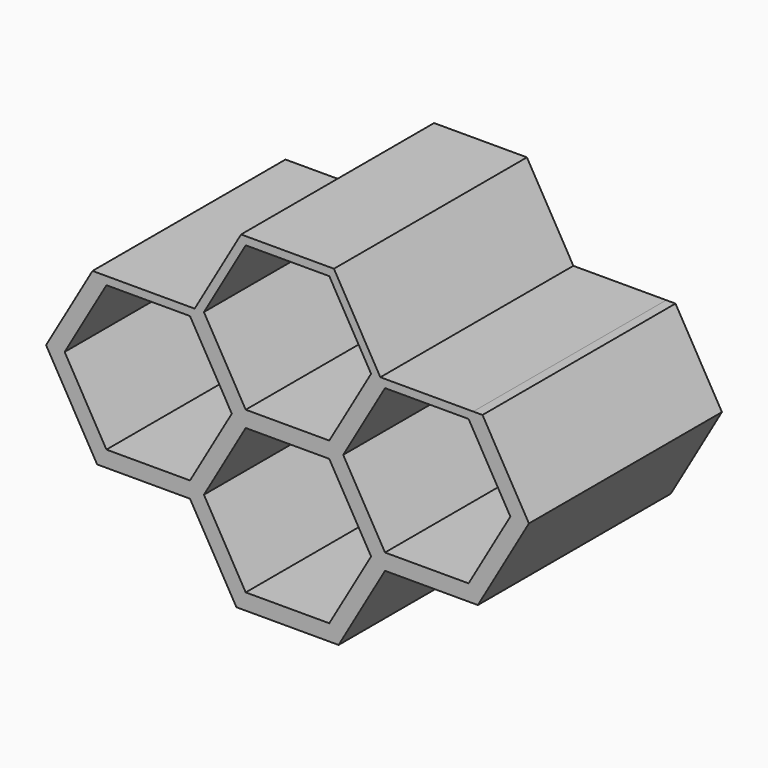
from build123d import *

# Parameters (mm, degrees)
F1_DEPTH = 12.7
F2_DEPTH = 95.25


# Not quite as in the source:
# - a feature names something its author has since deleted; it is built from what else it names


with BuildPart() as f1:
    # F0 (on Front) → F1 (new body)
    with BuildSketch(Plane.XZ):
        Polygon((142.3687008922, 35.0424993012), (105.7069587986, 35.0424993011), (87.3760877519, 3.2924993012), (105.7069587986, -28.4575006988), (142.3687008922, -28.4575006988), (160.6995719389, 3.2924993012), align=None)
        Polygon((107.5400459033, -25.2825006989), (91.0422619612, 3.2924993011), (107.5400459033, 31.8674993011), (140.5356137875, 31.8674993012), (157.0333977296, 3.2924993012), (140.5356137875, -25.2825006988), align=None, mode=Mode.SUBTRACT)
        Polygon((105.7069587986, -28.4575006988), (87.3760877519, 3.2924993012), (50.7143456583, 3.2924993012), (32.3834746115, -28.4575006988), (50.7143456583, -60.2075006988), (87.3760877519, -60.2075006988), align=None)
        Polygon((52.547432763, -57.0325006988), (36.0496488209, -28.4575006988), (52.547432763, 0.1174993012), (85.5430006472, 0.1174993012), (102.0407845893, -28.4575006988), (85.5430006472, -57.0325006988), align=None, mode=Mode.SUBTRACT)
        Polygon((197.3613140325, 3.2924993012), (160.6995719389, 3.2924993012), (142.3687008922, -28.4575006988), (160.6995719389, -60.2075006988), (197.3613140325, -60.2075006988), (215.6921850793, -28.4575006988), align=None)
        Polygon((162.5326590436, -57.0325006988), (146.0348751015, -28.4575006988), (162.5326590436, 0.1174993012), (195.5282269278, 0.1174993012), (212.0260108699, -28.4575006988), (195.5282269278, -57.0325006988), align=None, mode=Mode.SUBTRACT)
        Polygon((142.3687008922, -28.4575006988), (105.7069587986, -28.4575006989), (87.3760877519, -60.2075006988), (105.7069587986, -91.9575006988), (142.3687008922, -91.9575006988), (160.6995719389, -60.2075006988), align=None)
        Polygon((107.5400459033, -88.7825006988), (91.0422619612, -60.2075006988), (107.5400459033, -31.6325006988), (140.5356137875, -31.6325006988), (157.0333977296, -60.2075006988), (140.5356137875, -88.7825006988), align=None, mode=Mode.SUBTRACT)
        Polygon((162.5326590436, 0.1174993012), (146.0348751015, -28.4575006988), (162.5326590436, -57.0325006988), (195.5282269278, -57.0325006988), (212.0260108699, -28.4575006988), (195.5282269278, 0.1174993012), align=None)
        Polygon((52.547432763, 0.1174993012), (36.0496488209, -28.4575006988), (52.547432763, -57.0325006988), (85.5430006472, -57.0325006988), (102.0407845893, -28.4575006988), (85.5430006472, 0.1174993012), align=None)
        Polygon((107.5400459033, 31.8674993011), (91.0422619612, 3.2924993011), (107.5400459033, -25.2825006989), (140.5356137875, -25.2825006988), (157.0333977296, 3.2924993012), (140.5356137875, 31.8674993012), align=None)
        Polygon((107.5400459033, -31.6325006988), (91.0422619612, -60.2075006988), (107.5400459033, -88.7825006988), (140.5356137875, -88.7825006988), (157.0333977296, -60.2075006988), (140.5356137875, -31.6325006988), align=None)
    extrude(amount=F1_DEPTH)

    # F0 (on Front) → F2 (join)
    with BuildSketch(Plane.XZ):
        Polygon((142.3687008922, 35.0424993012), (105.7069587986, 35.0424993011), (87.3760877519, 3.2924993012), (105.7069587986, -28.4575006988), (142.3687008922, -28.4575006988), (160.6995719389, 3.2924993012), align=None)
        Polygon((107.5400459033, -25.2825006989), (91.0422619612, 3.2924993011), (107.5400459033, 31.8674993011), (140.5356137875, 31.8674993012), (157.0333977296, 3.2924993012), (140.5356137875, -25.2825006988), align=None, mode=Mode.SUBTRACT)
        Polygon((197.3613140325, 3.2924993012), (160.6995719389, 3.2924993012), (142.3687008922, -28.4575006988), (160.6995719389, -60.2075006988), (197.3613140325, -60.2075006988), (215.6921850793, -28.4575006988), align=None)
        Polygon((162.5326590436, -57.0325006988), (146.0348751015, -28.4575006988), (162.5326590436, 0.1174993012), (195.5282269278, 0.1174993012), (212.0260108699, -28.4575006988), (195.5282269278, -57.0325006988), align=None, mode=Mode.SUBTRACT)
        Polygon((142.3687008922, -28.4575006988), (105.7069587986, -28.4575006989), (87.3760877519, -60.2075006988), (105.7069587986, -91.9575006988), (142.3687008922, -91.9575006988), (160.6995719389, -60.2075006988), align=None)
        Polygon((107.5400459033, -88.7825006988), (91.0422619612, -60.2075006988), (107.5400459033, -31.6325006988), (140.5356137875, -31.6325006988), (157.0333977296, -60.2075006988), (140.5356137875, -88.7825006988), align=None, mode=Mode.SUBTRACT)
        Polygon((105.7069587986, -28.4575006988), (87.3760877519, 3.2924993012), (50.7143456583, 3.2924993012), (32.3834746115, -28.4575006988), (50.7143456583, -60.2075006988), (87.3760877519, -60.2075006988), align=None)
        Polygon((52.547432763, -57.0325006988), (36.0496488209, -28.4575006988), (52.547432763, 0.1174993012), (85.5430006472, 0.1174993012), (102.0407845893, -28.4575006988), (85.5430006472, -57.0325006988), align=None, mode=Mode.SUBTRACT)
        Polygon((32.3834746115, -28.4575006988), (50.7143456583, 3.2924993012), (47.048171449, 3.2924993012), (28.7173004022, -28.4575006988), (48.8812585536, -63.3825006988), (85.5430006472, -63.3825006988), (103.873871694, -95.1325006988), (144.2017879969, -95.1325006988), (162.5326590436, -63.3825006988), (199.1944011372, -63.3825006988), (219.3583592886, -28.4575006988), (201.0274882418, 3.2924993011), (197.3613140325, 3.2924993012), (215.6921850793, -28.4575006988), (197.3613140325, -60.2075006988), (160.6995719389, -60.2075006988), (142.3687008922, -91.9575006988), (105.7069587986, -91.9575006988), (87.3760877519, -60.2075006988), (50.7143456583, -60.2075006988), align=None)
    extrude(amount=F2_DEPTH)


solid = f1.part
